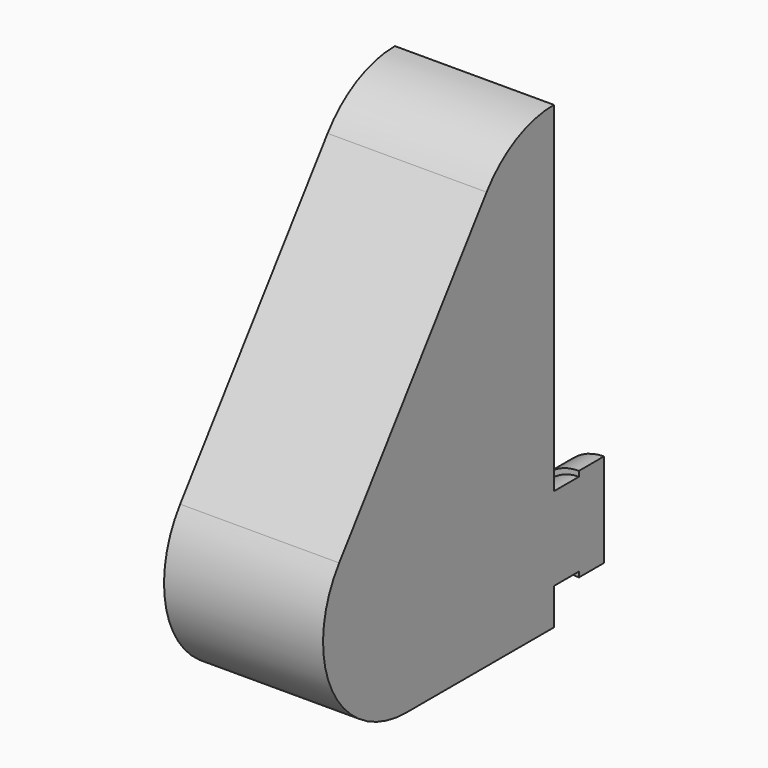
from build123d import *

# Parameters (mm, degrees)
F1_DEPTH    = 15.25
F2_T1_DEPTH = 107.2974570989
F3_W        = 3
F3_H        = 4
F4_ANGLE    = 180


# Not quite as in the source:
# - a fillet or chamfer that OpenCascade refuses, or shapes differently, is made with other operations: its cross-section is extruded or revolved along the edge and cut away or added


with BuildPart() as f1:
    # F0 (on Right) → F1 (new body)
    with BuildSketch(Plane.YZ):
        with BuildLine():
            Line((27.3567325823, 33.1807983013), (27.3567325823, 43.1807983013))
            ThreePointArc((27.3567325823, 43.1807983013), (22.8348355324, 42.1000161521), (19.2903756049, 39.0912877154))
            Line((19.2903756049, 39.0912877154), (27.3567325823, 33.1807983013))
        make_face()
        with BuildLine():
            Line((27.3567325823, 23.1807983013), (27.3567325823, 33.1807983013))
            Line((27.3567325823, 33.1807983013), (21.4462431681, 25.1144413239))
            ThreePointArc((21.4462431681, 25.1144413239), (24.2473572248, 23.6764948083), (27.3567325823, 23.1807983013))
        make_face()
        with BuildLine():
            Line((21.4462431681, 25.1144413239), (27.3567325823, 33.1807983013))
            Line((27.3567325823, 33.1807983013), (19.2903756049, 39.0912877154))
            ThreePointArc((19.2903756049, 39.0912877154), (17.4736097193, 31.656369728), (21.4462431681, 25.1144413239))
        make_face()
        with BuildLine():
            ThreePointArc((21.4462431681, 25.1144413239), (17.4736097193, 31.656369728), (19.2903756049, 39.0912877154))
            Line((19.2903756049, 39.0912877154), (-5.7096243951, 4.9724677154))
            ThreePointArc((-5.7096243951, 4.9724677154), (0.832304009, 8.9451011642), (8.2672219964, 7.1283352786))
            Line((8.2672219964, 7.1283352786), (21.4462431681, 25.1144413239))
        make_face()
        with BuildLine():
            ThreePointArc((-5.7096243951, 4.9724677154), (-7.1475709107, 2.1713536587), (-7.6432674177, -0.9380216987))
            Line((-7.6432674177, -0.9380216987), (2.3567325823, -0.9380216987))
            Line((2.3567325823, -0.9380216987), (-5.7096243951, 4.9724677154))
        make_face()
        with BuildLine():
            Line((27.3567325823, -0.9380216987), (27.3567325823, 23.1807983013))
            ThreePointArc((27.3567325823, 23.1807983013), (24.2473572248, 23.6764948083), (21.4462431681, 25.1144413239))
            Line((21.4462431681, 25.1144413239), (8.2672219964, 7.1283352786))
            ThreePointArc((8.2672219964, 7.1283352786), (11.2759504331, 3.5838753511), (12.3567325823, -0.9380216987))
            Line((12.3567325823, -0.9380216987), (27.3567325823, -0.9380216987))
        make_face()
        with BuildLine():
            ThreePointArc((8.2672219964, 7.1283352786), (0.832304009, 8.9451011642), (-5.7096243951, 4.9724677154))
            Line((-5.7096243951, 4.9724677154), (2.3567325823, -0.9380216987))
            Line((2.3567325823, -0.9380216987), (8.2672219964, 7.1283352786))
        make_face()
        with BuildLine():
            Line((8.2672219964, 7.1283352786), (2.3567325823, -0.9380216987))
            Line((2.3567325823, -0.9380216987), (12.3567325823, -0.9380216987))
            ThreePointArc((12.3567325823, -0.9380216987), (11.2759504331, 3.5838753511), (8.2672219964, 7.1283352786))
        make_face()
    extrude(amount=F1_DEPTH)

    # F2: fillet of radius 10 on 1 edges, made by hand

    # F2_s2 → F2_t1 (cut)
    with BuildSketch(Plane.YZ.offset(-46.0237285495)):
        with BuildLine():
            ThreePointArc((1.6177099031, 14.9724677154), (0.7648490296, 4.5400812514), (9.6840668804, -0.9380216987))
            Line((9.6840668804, -0.9380216987), (9.6840668804, -1.9380216987))
            Line((9.6840668804, -1.9380216987), (-7.6432674177, -1.9380216987))
            Line((-7.6432674177, -1.9380216987), (-8.6432674177, -0.9380216987))
            ThreePointArc((-8.6432674177, -0.9380216987), (-6.5162600928, 5.5635166568), (0.8110742054, 15.5635166568))
            Line((0.8110742054, 15.5635166568), (1.6177099031, 14.9724677154))
        make_face()
    extrude(amount=F2_T1_DEPTH, mode=Mode.SUBTRACT)

    # F3 (on face) → F4 (revolve)
    with BuildSketch(Plane.YZ.offset(15.25)):
        with Locations((28.8567325823, 4.5619783013)):
            Rectangle(F3_W, F3_H)
        Polygon((33.3567325823, 6.5619783013), (30.3567325823, 6.5619783013), (30.3567325823, 2.5619783013), (30.3567325823, 2.0619783013), (33.3567325823, 2.0619783013), align=None)
    revolve(axis=Axis((15.25, 28.8567325823, 6.5619783013), (0, 1, 0)), revolution_arc=F4_ANGLE)


solid = f1.part
